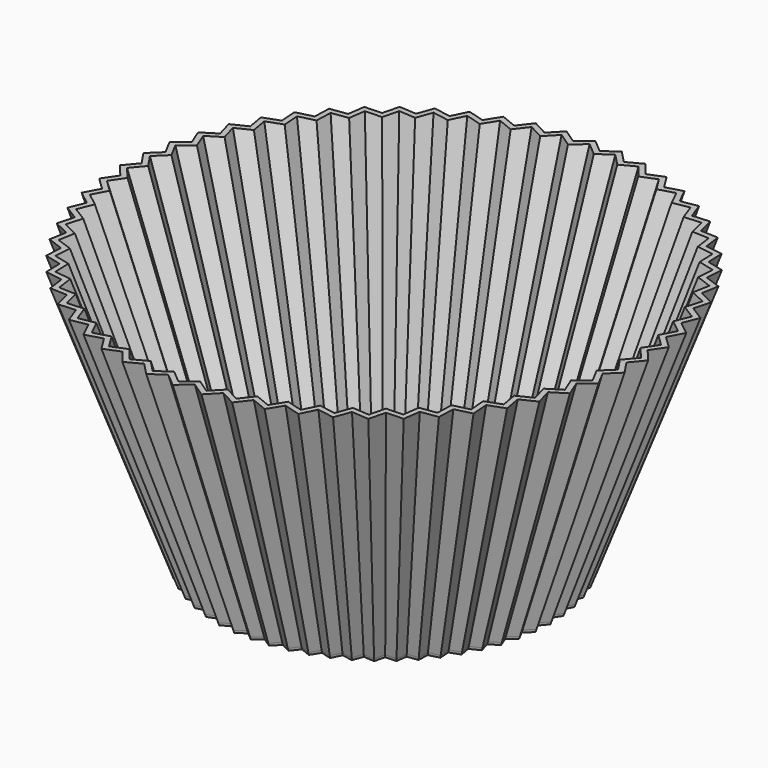
from build123d import *

# Parameters (mm, degrees)
F5_W      = 114.2538525164
F5_H      = 123.2350692153
F6_DEPTH  = 25.4
F11_DEPTH = 0.79375
F11_TAPER = 16


with BuildPart() as f3:
    # F0 (on Top) → F3 section 0
    with BuildSketch(Plane.XY):
        Polygon((7.965068901, 75.7825684271), (3.8252558243, 72.9902292487), (0, 76.2), (-3.8252558243, 72.9902292487), (-7.965068901, 75.7825684271), (-11.4338571696, 72.1905330228), (-15.8428708403, 74.5348471759), (-18.917186783, 70.5999022104), (-23.5470949714, 72.4705065417), (-26.1932557393, 68.2357640953), (-30.9933322024, 69.6121638724), (-33.1823459045, 65.1240206696), (-38.1, 65.9911357684), (-39.8078833441, 61.2987648453), (-44.7892362247, 61.6470949714), (-45.9972772835, 56.8019069257), (-50.9877522045, 56.6276357014), (-51.6827154274, 51.6827154274), (-56.6276357014, 50.9877522045), (-56.8019069257, 45.9972772835), (-61.6470949714, 44.7892362247), (-61.2987648453, 39.8078833441), (-65.9911357684, 38.1), (-65.1240206696, 33.1823459045), (-69.6121638724, 30.9933322024), (-68.2357640953, 26.1932557393), (-72.4705065417, 23.5470949714), (-70.5999022104, 18.917186783), (-74.5348471759, 15.8428708403), (-72.1905330228, 11.4338571696), (-75.7825684271, 7.965068901), (-72.9902292487, 3.8252558243), (-76.2, 0), (-72.9902292487, -3.8252558243), (-75.7825684271, -7.965068901), (-72.1905330228, -11.4338571696), (-74.5348471759, -15.8428708403), (-70.5999022104, -18.917186783), (-72.4705065417, -23.5470949714), (-68.2357640953, -26.1932557393), (-69.6121638724, -30.9933322024), (-65.1240206696, -33.1823459045), (-65.9911357684, -38.1), (-61.2987648453, -39.8078833441), (-61.6470949714, -44.7892362247), (-56.8019069257, -45.9972772835), (-56.6276357014, -50.9877522045), (-51.6827154274, -51.6827154274), (-50.9877522045, -56.6276357014), (-45.9972772835, -56.8019069257), (-44.7892362247, -61.6470949714), (-39.8078833441, -61.2987648453), (-38.1, -65.9911357684), (-33.1823459045, -65.1240206696), (-30.9933322024, -69.6121638724), (-26.1932557393, -68.2357640953), (-23.5470949714, -72.4705065417), (-18.917186783, -70.5999022104), (-15.8428708403, -74.5348471759), (-11.4338571696, -72.1905330228), (-7.965068901, -75.7825684271), (-3.8252558243, -72.9902292487), (0, -76.2), (3.8252558243, -72.9902292487), (7.965068901, -75.7825684271), (11.4338571696, -72.1905330228), (15.8428708403, -74.5348471759), (18.917186783, -70.5999022104), (23.5470949714, -72.4705065417), (26.1932557393, -68.2357640953), (30.9933322024, -69.6121638724), (33.1823459045, -65.1240206696), (38.1, -65.9911357684), (39.8078833441, -61.2987648453), (44.7892362247, -61.6470949714), (45.9972772835, -56.8019069257), (50.9877522045, -56.6276357014), (51.6827154274, -51.6827154274), (56.6276357014, -50.9877522045), (56.8019069257, -45.9972772835), (61.6470949714, -44.7892362247), (61.2987648453, -39.8078833441), (65.9911357684, -38.1), (65.1240206696, -33.1823459045), (69.6121638724, -30.9933322024), (68.2357640953, -26.1932557393), (72.4705065417, -23.5470949714), (70.5999022104, -18.917186783), (74.5348471759, -15.8428708403), (72.1905330228, -11.4338571696), (75.7825684271, -7.965068901), (72.9902292487, -3.8252558243), (76.2, 0), (72.9902292487, 3.8252558243), (75.7825684271, 7.965068901), (72.1905330228, 11.4338571696), (74.5348471759, 15.8428708403), (70.5999022104, 18.917186783), (72.4705065417, 23.5470949714), (68.2357640953, 26.1932557393), (69.6121638724, 30.9933322024), (65.1240206696, 33.1823459045), (65.9911357684, 38.1), (61.2987648453, 39.8078833441), (61.6470949714, 44.7892362247), (56.8019069257, 45.9972772835), (56.6276357014, 50.9877522045), (51.6827154274, 51.6827154274), (50.9877522045, 56.6276357014), (45.9972772835, 56.8019069257), (44.7892362247, 61.6470949714), (39.8078833441, 61.2987648453), (38.1, 65.9911357684), (33.1823459045, 65.1240206696), (30.9933322024, 69.6121638724), (26.1932557393, 68.2357640953), (23.5470949714, 72.4705065417), (18.917186783, 70.5999022104), (15.8428708403, 74.5348471759), (11.4338571696, 72.1905330228), align=None)
    # F2 (on offset) → F3 section 1
    with BuildSketch(Plane.XY.offset(-76.2)):
        Polygon((5.0179934076, 47.743018109), (2.4099111693, 45.9838444267), (0, 48.006), (-2.4099111693, 45.9838444267), (-5.0179934076, 47.743018109), (-7.2033300168, 45.4800358044), (-9.9810086294, 46.9569537208), (-11.9178276733, 44.4779383925), (-14.834669832, 45.6564191213), (-16.5017511158, 42.98853138), (-19.5257992875, 43.8556632396), (-20.9048779199, 41.0281330218), (-24.003, 41.5744155341), (-25.0789665068, 38.6182218525), (-28.2172188216, 38.837669832), (-28.9782846886, 35.7852013632), (-32.1222838889, 35.6754104919), (-32.5601107193, 32.5601107193), (-35.6754104919, 32.1222838889), (-35.7852013632, 28.9782846886), (-38.837669832, 28.2172188216), (-38.6182218525, 25.0789665068), (-41.5744155341, 24.003), (-41.0281330218, 20.9048779199), (-43.8556632396, 19.5257992875), (-42.98853138, 16.5017511158), (-45.6564191213, 14.834669832), (-44.4779383925, 11.9178276733), (-46.9569537208, 9.9810086294), (-45.4800358044, 7.2033300168), (-47.743018109, 5.0179934076), (-45.9838444267, 2.4099111693), (-48.006, 0), (-45.9838444267, -2.4099111693), (-47.743018109, -5.0179934076), (-45.4800358044, -7.2033300168), (-46.9569537208, -9.9810086294), (-44.4779383925, -11.9178276733), (-45.6564191213, -14.834669832), (-42.98853138, -16.5017511158), (-43.8556632396, -19.5257992875), (-41.0281330218, -20.9048779199), (-41.5744155341, -24.003), (-38.6182218525, -25.0789665068), (-38.837669832, -28.2172188216), (-35.7852013632, -28.9782846886), (-35.6754104919, -32.1222838889), (-32.5601107193, -32.5601107193), (-32.1222838889, -35.6754104919), (-28.9782846886, -35.7852013632), (-28.2172188216, -38.837669832), (-25.0789665068, -38.6182218525), (-24.003, -41.5744155341), (-20.9048779199, -41.0281330218), (-19.5257992875, -43.8556632396), (-16.5017511158, -42.98853138), (-14.834669832, -45.6564191213), (-11.9178276733, -44.4779383925), (-9.9810086294, -46.9569537208), (-7.2033300168, -45.4800358044), (-5.0179934076, -47.743018109), (-2.4099111693, -45.9838444267), (0, -48.006), (2.4099111693, -45.9838444267), (5.0179934076, -47.743018109), (7.2033300168, -45.4800358044), (9.9810086294, -46.9569537208), (11.9178276733, -44.4779383925), (14.834669832, -45.6564191213), (16.5017511158, -42.98853138), (19.5257992875, -43.8556632396), (20.9048779199, -41.0281330218), (24.003, -41.5744155341), (25.0789665068, -38.6182218525), (28.2172188216, -38.837669832), (28.9782846886, -35.7852013632), (32.1222838889, -35.6754104919), (32.5601107193, -32.5601107193), (35.6754104919, -32.1222838889), (35.7852013632, -28.9782846886), (38.837669832, -28.2172188216), (38.6182218525, -25.0789665068), (41.5744155341, -24.003), (41.0281330218, -20.9048779199), (43.8556632396, -19.5257992875), (42.98853138, -16.5017511158), (45.6564191213, -14.834669832), (44.4779383925, -11.9178276733), (46.9569537208, -9.9810086294), (45.4800358044, -7.2033300168), (47.743018109, -5.0179934076), (45.9838444267, -2.4099111693), (48.006, 0), (45.9838444267, 2.4099111693), (47.743018109, 5.0179934076), (45.4800358044, 7.2033300168), (46.9569537208, 9.9810086294), (44.4779383925, 11.9178276733), (45.6564191213, 14.834669832), (42.98853138, 16.5017511158), (43.8556632396, 19.5257992875), (41.0281330218, 20.9048779199), (41.5744155341, 24.003), (38.6182218525, 25.0789665068), (38.837669832, 28.2172188216), (35.7852013632, 28.9782846886), (35.6754104919, 32.1222838889), (32.5601107193, 32.5601107193), (32.1222838889, 35.6754104919), (28.9782846886, 35.7852013632), (28.2172188216, 38.837669832), (25.0789665068, 38.6182218525), (24.003, 41.5744155341), (20.9048779199, 41.0281330218), (19.5257992875, 43.8556632396), (16.5017511158, 42.98853138), (14.834669832, 45.6564191213), (11.9178276733, 44.4779383925), (9.9810086294, 46.9569537208), (7.2033300168, 45.4800358044), align=None)
    loft()

    # F5 (on offset) → F6 (cut)
    with BuildSketch(Plane.XY.offset(-75.40625)):
        with Locations((0.0083204359, -5.9572048485)):
            Rectangle(F5_W, F5_H)
    extrude(amount=-F6_DEPTH, mode=Mode.SUBTRACT)

    # F7 (on face) → F9 section 0
    with BuildSketch(Plane(origin=(0, 0, -75.40625), x_dir=(1, 0, 0), z_dir=(0, 0, -1))):
        Polygon((-2.320622742, 44.2801197412), (-4.8320742148, 45.9741151493), (-6.9364429977, 43.7949774832), (-9.6112072133, 45.2171748441), (-11.4762661323, 42.8300082871), (-14.2850378143, 43.964825709), (-15.8903528937, 41.3957845574), (-18.8023585517, 42.2307887432), (-20.1303416234, 39.5080199496), (-23.1136767141, 40.0340624185), (-24.1497781178, 37.1873972075), (-27.1717565976, 37.3987145284), (-27.9046245895, 34.4593415597), (-30.9321370298, 34.3536184957), (-31.3537421547, 31.3537421547), (-34.3536184957, 30.9321370298), (-34.4593415597, 27.9046245895), (-37.3987145284, 27.1717565976), (-37.1873972075, 24.1497781178), (-40.0340624185, 23.1136767141), (-39.5080199496, 20.1303416234), (-42.2307887432, 18.8023585517), (-41.3957845574, 15.8903528937), (-43.964825709, 14.2850378143), (-42.8300082871, 11.4762661323), (-45.2171748441, 9.6112072133), (-43.7949774832, 6.9364429977), (-45.9741151493, 4.8320742148), (-44.2801197412, 2.320622742), (-46.2273534282, 0), (-44.2801197412, -2.320622742), (-45.9741151493, -4.8320742148), (-43.7949774832, -6.9364429977), (-45.2171748441, -9.6112072133), (-42.8300082871, -11.4762661323), (-43.964825709, -14.2850378143), (-41.3957845574, -15.8903528937), (-42.2307887432, -18.8023585517), (-39.5080199496, -20.1303416234), (-40.0340624185, -23.1136767141), (-37.1873972075, -24.1497781178), (-37.3987145284, -27.1717565976), (-34.4593415597, -27.9046245895), (-34.3536184957, -30.9321370298), (-31.3537421547, -31.3537421547), (-30.9321370298, -34.3536184957), (-27.9046245895, -34.4593415597), (-27.1717565976, -37.3987145284), (-24.1497781178, -37.1873972075), (-23.1136767141, -40.0340624185), (-20.1303416234, -39.5080199496), (-18.8023585517, -42.2307887432), (-15.8903528937, -41.3957845574), (-14.2850378143, -43.964825709), (-11.4762661323, -42.8300082871), (-9.6112072133, -45.2171748441), (-6.9364429977, -43.7949774832), (-4.8320742148, -45.9741151493), (-2.320622742, -44.2801197412), (0, -46.2273534282), (2.320622742, -44.2801197412), (4.8320742148, -45.9741151493), (6.9364429977, -43.7949774832), (9.6112072133, -45.2171748441), (11.4762661323, -42.8300082871), (14.2850378143, -43.964825709), (15.8903528937, -41.3957845574), (18.8023585517, -42.2307887432), (20.1303416234, -39.5080199496), (23.1136767141, -40.0340624185), (24.1497781178, -37.1873972075), (27.1717565976, -37.3987145284), (27.9046245895, -34.4593415597), (30.9321370298, -34.3536184957), (31.3537421547, -31.3537421547), (34.3536184957, -30.9321370298), (34.4593415597, -27.9046245895), (37.3987145284, -27.1717565976), (37.1873972075, -24.1497781178), (40.0340624185, -23.1136767141), (39.5080199496, -20.1303416234), (42.2307887432, -18.8023585517), (41.3957845574, -15.8903528937), (43.964825709, -14.2850378143), (42.8300082871, -11.4762661323), (45.2171748441, -9.6112072133), (43.7949774832, -6.9364429977), (45.9741151493, -4.8320742148), (44.2801197412, -2.320622742), (46.2273534282, 0), (44.2801197412, 2.320622742), (45.9741151493, 4.8320742148), (43.7949774832, 6.9364429977), (45.2171748441, 9.6112072133), (42.8300082871, 11.4762661323), (43.964825709, 14.2850378143), (41.3957845574, 15.8903528937), (42.2307887432, 18.8023585517), (39.5080199496, 20.1303416234), (40.0340624185, 23.1136767141), (37.1873972075, 24.1497781178), (37.3987145284, 27.1717565976), (34.4593415597, 27.9046245895), (34.3536184957, 30.9321370298), (31.3537421547, 31.3537421547), (30.9321370298, 34.3536184957), (27.9046245895, 34.4593415597), (27.1717565976, 37.3987145284), (24.1497781178, 37.1873972075), (23.1136767141, 40.0340624185), (20.1303416234, 39.5080199496), (18.8023585517, 42.2307887432), (15.8903528937, 41.3957845574), (14.2850378143, 43.964825709), (11.4762661323, 42.8300082871), (9.6112072133, 45.2171748441), (6.9364429977, 43.7949774832), (4.8320742148, 45.9741151493), (2.320622742, 44.2801197412), (0, 46.2273534282), align=None)
    # F8 (on face) → F9 section 1
    with BuildSketch(Plane.XY):
        Polygon((-55.0875913592, -49.6010900505), (-50.2771530638, -50.2771530638), (-49.6010900505, -55.0875913592), (-44.7463360115, -55.257123106), (-43.5711488195, -59.9705414893), (-38.7252687381, -59.6316845441), (-37.0638329641, -64.1964418171), (-32.2799193166, -63.3529087676), (-30.1504379987, -67.7189924943), (-25.4809043441, -66.3800252652), (-22.9067085252, -70.4995997188), (-18.4027152513, -68.6798683151), (-15.4120083595, -72.5077985757), (-11.1229021593, -70.2272403556), (-7.7484510051, -73.7215868181), (-3.7212242235, -71.0051880547), (0, -74.1276659282), (3.7212242235, -71.0051880547), (7.7484510051, -73.7215868181), (11.1229021593, -70.2272403556), (15.4120083595, -72.5077985757), (18.4027152513, -68.6798683151), (22.9067085252, -70.4995997188), (25.4809043441, -66.3800252652), (30.1504379987, -67.7189924943), (32.2799193166, -63.3529087676), (37.0638329641, -64.1964418171), (38.7252687381, -59.6316845441), (43.5711488195, -59.9705414893), (44.7463360115, -55.257123106), (49.6010900505, -55.0875913592), (50.2771530638, -50.2771530638), (55.0875913592, -49.6010900505), (55.257123106, -44.7463360115), (59.9705414893, -43.5711488195), (59.6316845441, -38.7252687381), (64.1964418171, -37.0638329641), (63.3529087676, -32.2799193166), (67.7189924943, -30.1504379987), (66.3800252652, -25.4809043441), (70.4995997188, -22.9067085252), (68.6798683151, -18.4027152513), (72.5077985757, -15.4120083595), (70.2272403556, -11.1229021593), (73.7215868181, -7.7484510051), (71.0051880547, -3.7212242235), (74.1276659282, 0), (71.0051880547, 3.7212242235), (73.7215868181, 7.7484510051), (70.2272403556, 11.1229021593), (72.5077985757, 15.4120083595), (68.6798683151, 18.4027152513), (70.4995997188, 22.9067085252), (66.3800252652, 25.4809043441), (67.7189924943, 30.1504379987), (63.3529087676, 32.2799193166), (64.1964418171, 37.0638329641), (59.6316845441, 38.7252687381), (59.9705414893, 43.5711488195), (55.257123106, 44.7463360115), (55.0875913592, 49.6010900505), (50.2771530638, 50.2771530638), (49.6010900505, 55.0875913592), (44.7463360115, 55.257123106), (43.5711488195, 59.9705414893), (38.7252687381, 59.6316845441), (37.0638329641, 64.1964418171), (32.2799193166, 63.3529087676), (30.1504379987, 67.7189924943), (25.4809043441, 66.3800252652), (22.9067085252, 70.4995997188), (18.4027152513, 68.6798683151), (15.4120083595, 72.5077985757), (11.1229021593, 70.2272403556), (7.7484510051, 73.7215868181), (3.7212242235, 71.0051880547), (0, 74.1276659282), (-3.7212242235, 71.0051880547), (-7.7484510051, 73.7215868181), (-11.1229021593, 70.2272403556), (-15.4120083595, 72.5077985757), (-18.4027152513, 68.6798683151), (-22.9067085252, 70.4995997188), (-25.4809043441, 66.3800252652), (-30.1504379987, 67.7189924943), (-32.2799193166, 63.3529087676), (-37.0638329641, 64.1964418171), (-38.7252687381, 59.6316845441), (-43.5711488195, 59.9705414893), (-44.7463360115, 55.257123106), (-49.6010900505, 55.0875913592), (-50.2771530638, 50.2771530638), (-55.0875913592, 49.6010900505), (-55.257123106, 44.7463360115), (-59.9705414893, 43.5711488195), (-59.6316845441, 38.7252687381), (-64.1964418171, 37.0638329641), (-63.3529087676, 32.2799193166), (-67.7189924943, 30.1504379987), (-66.3800252652, 25.4809043441), (-70.4995997188, 22.9067085252), (-68.6798683151, 18.4027152513), (-72.5077985757, 15.4120083595), (-70.2272403556, 11.1229021593), (-73.7215868181, 7.7484510051), (-71.0051880547, 3.7212242235), (-74.1276659282, 0), (-71.0051880547, -3.7212242235), (-73.7215868181, -7.7484510051), (-70.2272403556, -11.1229021593), (-72.5077985757, -15.4120083595), (-68.6798683151, -18.4027152513), (-70.4995997188, -22.9067085252), (-66.3800252652, -25.4809043441), (-67.7189924943, -30.1504379987), (-63.3529087676, -32.2799193166), (-64.1964418171, -37.0638329641), (-59.6316845441, -38.7252687381), (-59.9705414893, -43.5711488195), (-55.257123106, -44.7463360115), align=None)
    loft(mode=Mode.SUBTRACT)

    # F10 (on face) → F11 (join)
    with BuildSketch(Plane(origin=(0, 0, -75.40625), x_dir=(1, 0, 0), z_dir=(0, 0, -1))):
        Polygon((-5.0486921107, 48.0350967582), (-7.247398008, 45.7582701504), (-10.0420696941, 47.2442234443), (-11.990737664, 44.7500421823), (-14.9254242605, 45.9357325319), (-16.602704289, 43.2515233875), (-19.6452527554, 44.1239601212), (-21.0327682114, 41.2791318515), (-24.14984375, 41.8287563698), (-25.2323927239, 38.8544775087), (-28.3898440028, 39.0752680105), (-29.1555658615, 36.0041253795), (-32.3187991838, 35.8936628378), (-32.7593045183, 32.7593045183), (-35.8936628378, 32.3187991838), (-36.0041253795, 29.1555658615), (-39.0752680105, 28.3898440028), (-38.8544775087, 25.2323927239), (-41.8287563698, 24.14984375), (-41.2791318515, 21.0327682114), (-44.1239601212, 19.6452527554), (-43.2515233875, 16.602704289), (-45.9357325319, 14.9254242605), (-44.7500421823, 11.990737664), (-47.2442234443, 10.0420696941), (-45.7582701504, 7.247398008), (-48.0350967582, 5.0486921107), (-46.2651609352, 2.4246543428), (-48.2996875, 0), (-46.2651609352, -2.4246543428), (-48.0350967582, -5.0486921107), (-45.7582701504, -7.247398008), (-47.2442234443, -10.0420696941), (-44.7500421823, -11.990737664), (-45.9357325319, -14.9254242605), (-43.2515233875, -16.602704289), (-44.1239601212, -19.6452527554), (-41.2791318515, -21.0327682114), (-41.8287563698, -24.14984375), (-38.8544775087, -25.2323927239), (-39.0752680105, -28.3898440028), (-36.0041253795, -29.1555658615), (-35.8936628378, -32.3187991838), (-32.7593045183, -32.7593045183), (-32.3187991838, -35.8936628378), (-29.1555658615, -36.0041253795), (-28.3898440028, -39.0752680105), (-25.2323927239, -38.8544775087), (-24.14984375, -41.8287563698), (-21.0327682114, -41.2791318515), (-19.6452527554, -44.1239601212), (-16.602704289, -43.2515233875), (-14.9254242605, -45.9357325319), (-11.990737664, -44.7500421823), (-10.0420696941, -47.2442234443), (-7.247398008, -45.7582701504), (-5.0486921107, -48.0350967582), (-2.4246543428, -46.2651609352), (0, -48.2996875), (2.4246543428, -46.2651609352), (5.0486921107, -48.0350967582), (7.247398008, -45.7582701504), (10.0420696941, -47.2442234443), (11.990737664, -44.7500421823), (14.9254242605, -45.9357325319), (16.602704289, -43.2515233875), (19.6452527554, -44.1239601212), (21.0327682114, -41.2791318515), (24.14984375, -41.8287563698), (25.2323927239, -38.8544775087), (28.3898440028, -39.0752680105), (29.1555658615, -36.0041253795), (32.3187991838, -35.8936628378), (32.7593045183, -32.7593045183), (35.8936628378, -32.3187991838), (36.0041253795, -29.1555658615), (39.0752680105, -28.3898440028), (38.8544775087, -25.2323927239), (41.8287563698, -24.14984375), (41.2791318515, -21.0327682114), (44.1239601212, -19.6452527554), (43.2515233875, -16.602704289), (45.9357325319, -14.9254242605), (44.7500421823, -11.990737664), (47.2442234443, -10.0420696941), (45.7582701504, -7.247398008), (48.0350967582, -5.0486921107), (46.2651609352, -2.4246543428), (48.2996875, 0), (46.2651609352, 2.4246543428), (48.0350967582, 5.0486921107), (45.7582701504, 7.247398008), (47.2442234443, 10.0420696941), (44.7500421823, 11.990737664), (45.9357325319, 14.9254242605), (43.2515233875, 16.602704289), (44.1239601212, 19.6452527554), (41.2791318515, 21.0327682114), (41.8287563698, 24.14984375), (38.8544775087, 25.2323927239), (39.0752680105, 28.3898440028), (36.0041253795, 29.1555658615), (35.8936628378, 32.3187991838), (32.7593045183, 32.7593045183), (32.3187991838, 35.8936628378), (29.1555658615, 36.0041253795), (28.3898440028, 39.0752680105), (25.2323927239, 38.8544775087), (24.14984375, 41.8287563698), (21.0327682114, 41.2791318515), (19.6452527554, 44.1239601212), (16.602704289, 43.2515233875), (14.9254242605, 45.9357325319), (11.990737664, 44.7500421823), (10.0420696941, 47.2442234443), (7.247398008, 45.7582701504), (5.0486921107, 48.0350967582), (2.4246543428, 46.2651609352), (0, 48.2996875), (-2.4246543428, 46.2651609352), align=None)
    extrude(amount=F11_DEPTH, taper=F11_TAPER)


solid = f3.part
